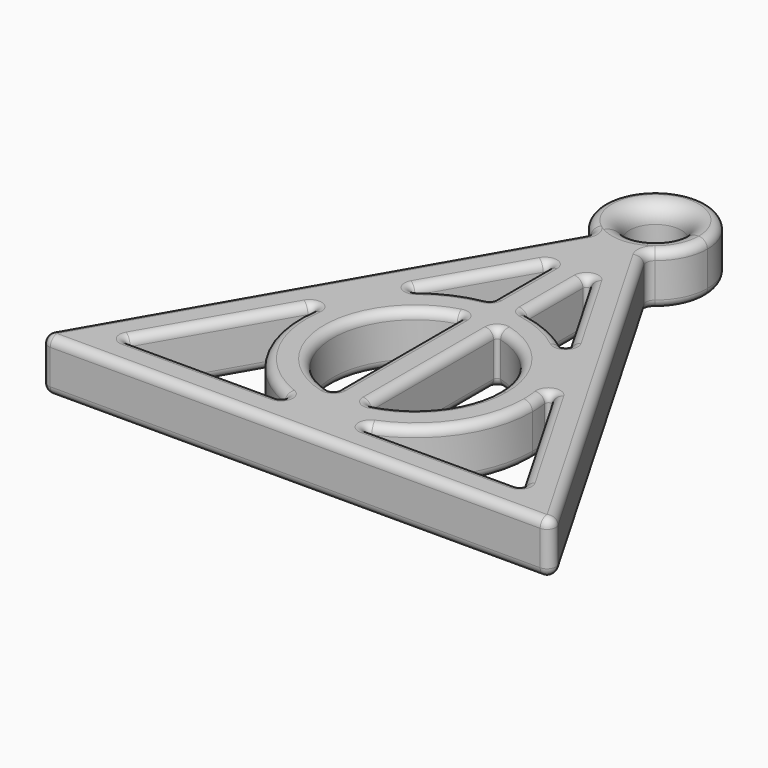
from build123d import *

# Parameters (mm, degrees)
F1_DEPTH = 1.5
F2_R     = 0.25
F3_R     = 0.25
F4_R     = 0.49999
F5_R     = 0.1
F6_R     = 0.25


# Not quite as in the source:
# - a fillet or chamfer is up to 0.001 mm smaller than in the source, because OpenCascade refuses the exact size


with BuildPart() as f1:
    # F0 (on Top) → F1 (new body)
    with BuildSketch(Plane.XY):
        with BuildLine():
            ThreePointArc((0.75, -1.2990381057), (0, -1.5), (-0.75, -1.2990381057))
            Line((-0.75, -1.2990381057), (-7.5, -12.9903810568))
            Line((-7.5, -12.9903810568), (7.5, -12.9903810568))
            Line((7.5, -12.9903810568), (0.75, -1.2990381057))
        make_face()
        with BuildLine():
            Line((-0.5, -2.8660254038), (0, -2))
            Line((0, -2), (0.5, -2.8660254038))
            Line((0.5, -2.8660254038), (2.5943573048, -6.4935586649))
            ThreePointArc((2.5943573048, -6.4935586649), (2.9272758664, -6.9701905284), (3.1735918876, -7.4968223918))
            Line((3.1735918876, -7.4968223918), (5.7679491924, -11.9903810568))
            Line((5.7679491924, -11.9903810568), (0.5792345828, -11.9903810568))
            ThreePointArc((0.5792345828, -11.9903810568), (0, -12.0403810568), (-0.5792345828, -11.9903810568))
            Line((-0.5792345828, -11.9903810568), (-5.7679491924, -11.9903810568))
            Line((-5.7679491924, -11.9903810568), (-3.1735918876, -7.4968223918))
            ThreePointArc((-3.1735918876, -7.4968223918), (-2.9272758664, -6.9701905284), (-2.5943573048, -6.4935586649))
            Line((-2.5943573048, -6.4935586649), (-0.5, -2.8660254038))
        make_face(mode=Mode.SUBTRACT)
        with BuildLine():
            ThreePointArc((-0.5, -5.3173124194), (-1.6551889892, -5.7131184668), (-2.5943573048, -6.4935586649))
            Line((-2.5943573048, -6.4935586649), (-3.1735918876, -7.4968223918))
            ThreePointArc((-3.1735918876, -7.4968223918), (-2.9272758664, -10.3503175473), (-0.5792345828, -11.9903810568))
            Line((-0.5792345828, -11.9903810568), (-0.5, -11.9903810568))
            Line((-0.5, -11.9903810568), (-0.5, -10.9872702875))
            ThreePointArc((-0.5, -10.9872702875), (-2.3801270189, -8.6602540378), (-0.5, -6.3332377882))
            Line((-0.5, -6.3332377882), (-0.5, -5.3173124194))
        make_face()
        with BuildLine():
            Line((3.1735918876, -7.4968223918), (2.5943573048, -6.4935586649))
            ThreePointArc((2.5943573048, -6.4935586649), (1.6551889892, -5.7131184668), (0.5, -5.3173124194))
            Line((0.5, -5.3173124194), (0.5, -6.3332377882))
            ThreePointArc((0.5, -6.3332377882), (1.8513600589, -7.164436349), (2.3801270189, -8.6602540378))
            ThreePointArc((2.3801270189, -8.6602540378), (1.8513600589, -10.1560717267), (0.5, -10.9872702875))
            Line((0.5, -10.9872702875), (0.5, -11.9903810568))
            Line((0.5, -11.9903810568), (0.5792345828, -11.9903810568))
            ThreePointArc((0.5792345828, -11.9903810568), (2.5868074076, -10.8359576252), (3.3801270189, -8.6602540378))
            ThreePointArc((3.3801270189, -8.6602540378), (3.3280927233, -8.0694431638), (3.1735918876, -7.4968223918))
        make_face()
        with BuildLine():
            ThreePointArc((0.5, -6.3332377882), (0, -6.2801270189), (-0.5, -6.3332377882))
            Line((-0.5, -6.3332377882), (-0.5, -10.9872702875))
            ThreePointArc((-0.5, -10.9872702875), (0, -11.0403810568), (0.5, -10.9872702875))
            Line((0.5, -10.9872702875), (0.5, -6.3332377882))
        make_face()
        with BuildLine():
            Line((-0.75, -1.2990381057), (-0.375, -0.6495190528))
            ThreePointArc((-0.375, -0.6495190528), (-0.375, 0.6495190528), (0.75, 0))
            ThreePointArc((0.75, 0), (0.6495190528, -0.375), (0.375, -0.6495190528))
            Line((0.375, -0.6495190528), (0.75, -1.2990381057))
            ThreePointArc((0.75, -1.2990381057), (1.2990381057, -0.75), (1.5, 0))
            ThreePointArc((1.5, 0), (-0.75, 1.2990381057), (-0.75, -1.2990381057))
        make_face()
        with BuildLine():
            Line((0.5, -2.8660254038), (0, -2))
            Line((0, -2), (-0.5, -2.8660254038))
            Line((-0.5, -2.8660254038), (-0.5, -5.3173124194))
            ThreePointArc((-0.5, -5.3173124194), (0, -5.2801270189), (0.5, -5.3173124194))
            Line((0.5, -5.3173124194), (0.5, -2.8660254038))
        make_face()
        with BuildLine():
            ThreePointArc((0.5, -5.3173124194), (0, -5.2801270189), (-0.5, -5.3173124194))
            Line((-0.5, -5.3173124194), (-0.5, -6.3332377882))
            ThreePointArc((-0.5, -6.3332377882), (0, -6.2801270189), (0.5, -6.3332377882))
            Line((0.5, -6.3332377882), (0.5, -5.3173124194))
        make_face()
        with BuildLine():
            ThreePointArc((0.5, -10.9872702875), (0, -11.0403810568), (-0.5, -10.9872702875))
            Line((-0.5, -10.9872702875), (-0.5, -11.9903810568))
            Line((-0.5, -11.9903810568), (0.5, -11.9903810568))
            Line((0.5, -11.9903810568), (0.5, -10.9872702875))
        make_face()
        with BuildLine():
            ThreePointArc((0.375, -0.6495190528), (0, -0.75), (-0.375, -0.6495190528))
            Line((-0.375, -0.6495190528), (-0.75, -1.2990381057))
            ThreePointArc((-0.75, -1.2990381057), (0, -1.5), (0.75, -1.2990381057))
            Line((0.75, -1.2990381057), (0.375, -0.6495190528))
        make_face()
        with BuildLine():
            Line((-0.5, -11.9903810568), (-0.5792345828, -11.9903810568))
            ThreePointArc((-0.5792345828, -11.9903810568), (0, -12.0403810568), (0.5792345828, -11.9903810568))
            Line((0.5792345828, -11.9903810568), (0.5, -11.9903810568))
            Line((0.5, -11.9903810568), (-0.5, -11.9903810568))
        make_face()
        with BuildLine():
            Line((-3.1735918876, -7.4968223918), (-2.5943573048, -6.4935586649))
            ThreePointArc((-2.5943573048, -6.4935586649), (-2.9272758664, -6.9701905284), (-3.1735918876, -7.4968223918))
        make_face()
        with BuildLine():
            ThreePointArc((3.1735918876, -7.4968223918), (2.9272758664, -6.9701905284), (2.5943573048, -6.4935586649))
            Line((2.5943573048, -6.4935586649), (3.1735918876, -7.4968223918))
        make_face()
    extrude(amount=F1_DEPTH)

    # F2
    f2_edges = [f1.edges().sort_by_distance(p)[0] for p in [
        (0.75, -1.299038, 0.75),
        (-0.75, -1.299038, 0.75),
        (-7.5, -12.990381, 0.75),
        (7.5, -12.990381, 0.75),
    ]]
    fillet(f2_edges, radius=F2_R)

    # F3
    f3_edges = [f1.edges().sort_by_distance(p)[0] for p in [
        (0, 1.5, 1.5),
        (0, 1.5, 0),
    ]]
    fillet(f3_edges, radius=F3_R)

    # F4 (radius 0.5 in the source; OpenCascade refuses exactly that, so slightly less here)
    f4_edges = [f1.edges().sort_by_distance(p)[0] for p in [
        (-0.75, 0, 1.5),
        (-0.75, 0, 0),
    ]]
    fillet(f4_edges, radius=F4_R)

    # F5
    f5_edges = [f1.edges().sort_by_distance(p)[0] for p in [
        (-0.5, -2.866025, 0.75),
        (-2.594357, -6.493559, 0.75),
        (-0.5, -5.317312, 0.75),
        (0.5, -2.866025, 0.75),
        (0.5, -5.317312, 0.75),
        (2.594357, -6.493559, 0.75),
        (5.767949, -11.990381, 0.75),
        (3.173592, -7.496822, 0.75),
        (-3.173592, -7.496822, 0.75),
        (-0.5, -6.333238, 0.75),
        (0.5, -6.333238, 0.75),
        (-0.5, -10.98727, 0.75),
        (-5.767949, -11.990381, 0.75),
        (0.5, -10.98727, 0.75),
        (0.579235, -11.990381, 0.75),
        (-0.579235, -11.990381, 0.75),
    ]]
    fillet(f5_edges, radius=F5_R)

    # F6
    f6_edges = [f1.edges().sort_by_distance(p)[0] for p in [
        (-1.461487, -4.531369, 1.5),
        (-1.461487, -4.531369, 0),
        (0.5, -4.235735, 1.5),
        (0.5, -4.235735, 0),
        (2.927276, -10.350318, 0),
        (0.5, -8.660254, 0),
        (-0.5, -8.660254, 0),
        (-2.927276, -10.350318, 0),
        (-2.927276, -10.350318, 1.5),
        (-0.5, -8.660254, 1.5),
        (0.5, -8.660254, 1.5),
        (2.927276, -10.350318, 1.5),
    ]]
    fillet(f6_edges, radius=F6_R)


solid = f1.part
